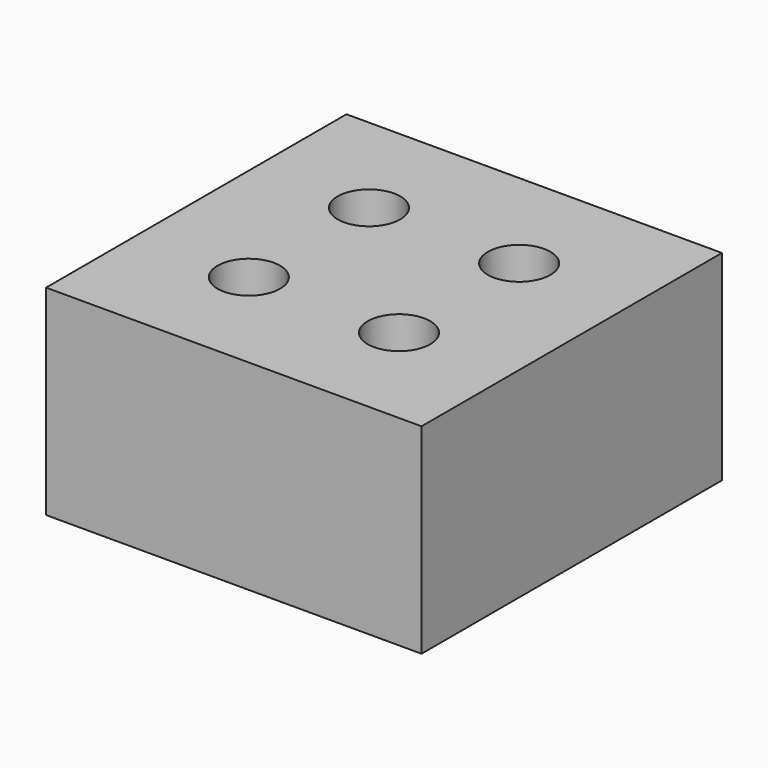
from build123d import *

# Parameters (mm, degrees)
F0_W     = 30
F0_H     = 30
F1_DEPTH = 16
F2_D     = 5


# Not quite as in the source:
# - a feature names something its author has since deleted; it is built from what else it names


with BuildPart() as f1:
    # F0 (on Top) → F1 (new body)
    with BuildSketch(Plane.XY):
        Rectangle(F0_W, F0_H)
    extrude(amount=F1_DEPTH)

    # F2 (through all)
    with Locations(Plane(origin=(0, 0, 0), x_dir=(1, 0, 0), z_dir=(0, 0, -1))):
        with Locations((-6, -6), (6, 6), (-6, 6), (6, -6)):
            Hole(F2_D / 2)


solid = f1.part
